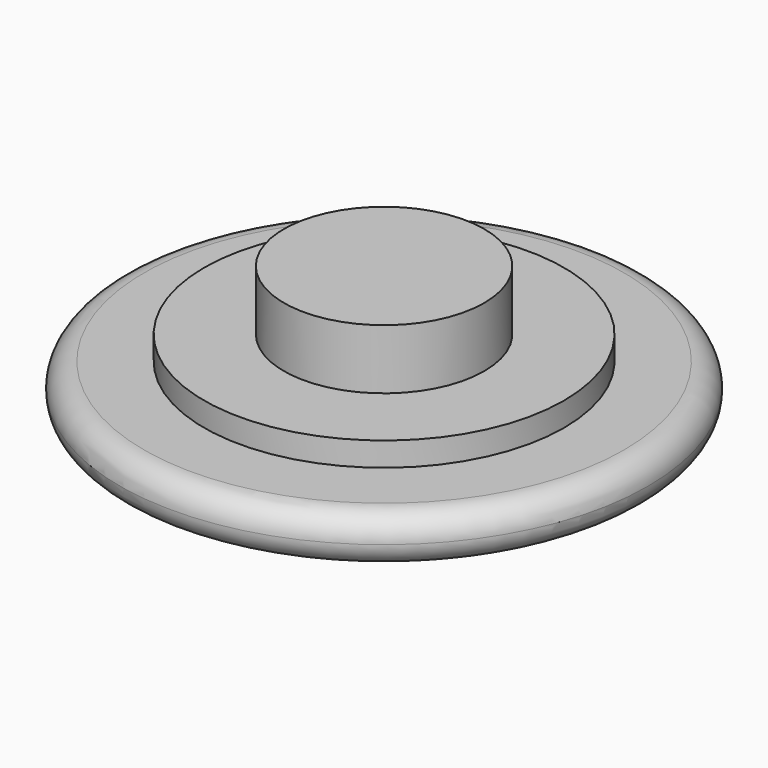
from build123d import *

# Parameters (mm, degrees)
F0_R         = 11
F0_R_2       = 7.5
F1_DEPTH     = 2
F0_R_3       = 4.175
F2_DEPTH     = 3
F3_DEPTH     = 5.5
F4_R         = 0.99999
F5_TEXT_SIZE = 9.9345928447
F6_DEPTH     = 1


# Not quite as in the source:
# - a fillet or chamfer is up to 0.001 mm smaller than in the source, because OpenCascade refuses the exact size
# - Text() gives the source's letters only with a copy of the font that has no kerning and outlines rounded to 1/6400 em; it was checked with that copy


with BuildPart() as f1:
    # F0 (on Top) → F1 (new body)
    with BuildSketch(Plane.XY):
        Circle(F0_R)
        Circle(F0_R_2, mode=Mode.SUBTRACT)
    extrude(amount=F1_DEPTH)

    # F0 (on Top) → F2 (join)
    with BuildSketch(Plane.XY):
        Circle(F0_R_2)
        Circle(F0_R_3, mode=Mode.SUBTRACT)
    extrude(amount=F2_DEPTH)

    # F0 (on Top) → F3 (join)
    with BuildSketch(Plane.XY):
        Circle(F0_R_3)
    extrude(amount=F3_DEPTH)

    # F4 (radius 1 in the source; OpenCascade refuses exactly that, so slightly less here)
    f4_edges = [f1.edges().sort_by_distance(p)[0] for p in [
        (-11, 0, 2),
        (-11, 0, 0),
    ]]
    fillet(f4_edges, radius=F4_R)

    # F5 (on face) → F6 (cut)
    with BuildSketch(Plane(origin=(0, 0, 0), x_dir=(1, 0, 0), z_dir=(0, 0, -1))):
        with Locations((-9.5161238905, -3.0730092906)):
            Text('Dad', F5_TEXT_SIZE, font='Open Sans', text_align=(TextAlign.LEFT, TextAlign.BOTTOM))
    extrude(amount=-F6_DEPTH, mode=Mode.SUBTRACT)


solid = f1.part
